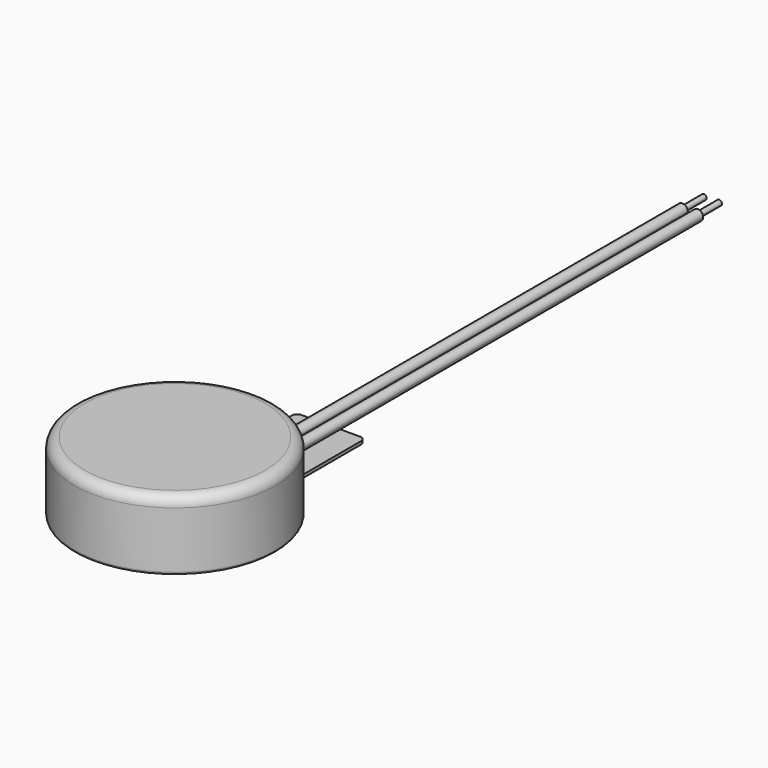
from build123d import *

# Parameters (mm, degrees)
F0_R      = 5.0038
F1_DEPTH  = 3.4544
F2_R      = 1.143
F3_DEPTH  = 0.1524
F6_DEPTH  = 1.27
F7_DEPTH  = 1.27
F8_DEPTH  = 27.94
F9_DEPTH  = 27.94
F10_R     = 0.2667
F10_R_2   = 0.13335
F11_DEPTH = 1.3335
F12_DEPTH = 1.3335
F13_R     = 0.508
F14_R     = 0.127


with BuildPart() as f1:
    # F0 (on Top) → F1 (new body)
    with BuildSketch(Plane.XY):
        with Locations((-16.2086095661, 14.8969562724)):
            Circle(F0_R)
    extrude(amount=F1_DEPTH)

    # F13
    f13_edges = [f1.edges().sort_by_distance(p)[0] for p in [
        (-21.21241, 14.896956, 3.4544),
    ]]
    fillet(f13_edges, radius=F13_R)

    # F14
    f14_edges = [f1.edges().sort_by_distance(p)[0] for p in [
        (-21.21241, 14.896956, 0),
    ]]
    fillet(f14_edges, radius=F14_R)


with BuildPart() as f3:
    # F2 (on face) → F3 (new body)
    with BuildSketch(Plane(origin=(0, 0, 0), x_dir=(1, 0, 0), z_dir=(0, 0, -1))):
        with BuildLine():
            Line((-17.9294595661, -19.2057716882), (-17.9294595661, -19.5955400716))
            ThreePointArc((-17.9294595661, -19.5955400716), (-16.2086095661, -19.9007562724), (-14.4877595661, -19.5955400716))
            Line((-14.4877595661, -19.5955400716), (-14.4877595661, -19.2057716882))
            ThreePointArc((-14.4877595661, -19.2057716882), (-14.3430605213, -18.6170461492), (-13.9419363215, -18.1624749774))
            ThreePointArc((-13.9419363215, -18.1624749774), (-16.2086095661, -10.9218562724), (-18.4752828106, -18.1624749774))
            ThreePointArc((-18.4752828106, -18.1624749774), (-18.0741586109, -18.6170461492), (-17.9294595661, -19.2057716882))
        make_face()
        with Locations((-16.2086095661, -14.8969562724)):
            Circle(F2_R, mode=Mode.SUBTRACT)
        with BuildLine():
            ThreePointArc((-14.4877595661, -19.5955400716), (-16.2086095661, -19.9007562724), (-17.9294595661, -19.5955400716))
            Line((-17.9294595661, -19.5955400716), (-17.9294595661, -24.3330562724))
            ThreePointArc((-17.9294595661, -24.3330562724), (-17.8550646885, -24.5126613948), (-17.6754595661, -24.5870562724))
            Line((-17.6754595661, -24.5870562724), (-14.7417595661, -24.5870562724))
            ThreePointArc((-14.7417595661, -24.5870562724), (-14.5621544437, -24.5126613948), (-14.4877595661, -24.3330562724))
            Line((-14.4877595661, -24.3330562724), (-14.4877595661, -19.5955400716))
        make_face()
    extrude(amount=F3_DEPTH)


with BuildPart() as f6:
    # F5 (on offset) → F6 (new body)
    with BuildSketch(Plane.XZ.offset(-20.32)):
        with BuildLine():
            ThreePointArc((-16.5896095661, 0), (-16.4010241876, 0.0781146215), (-16.3229095661, 0.2667))
            ThreePointArc((-16.3229095661, 0.2667), (-16.7781949446, 0.4552853785), (-16.5896095661, 0))
        make_face()
    extrude(amount=F6_DEPTH)

    # F5 (on offset) → F8 (join)
    with BuildSketch(Plane.XZ.offset(-20.32)):
        with BuildLine():
            ThreePointArc((-16.5896095661, 0), (-16.4010241876, 0.0781146215), (-16.3229095661, 0.2667))
            ThreePointArc((-16.3229095661, 0.2667), (-16.7781949446, 0.4552853785), (-16.5896095661, 0))
        make_face()
    extrude(amount=-F8_DEPTH)

    # F10 (on face) → F12 (cut)
    with BuildSketch(Plane(origin=(0, 48.26, 0), x_dir=(-1, 0, 0), z_dir=(0, 1, 0))):
        with Locations((16.5896095661, 0.2667)):
            Circle(F10_R)
        with Locations((16.5896095661, 0.2667)):
            Circle(F10_R_2, mode=Mode.SUBTRACT)
    extrude(amount=-F12_DEPTH, mode=Mode.SUBTRACT)


with BuildPart() as f7:
    # F5 (on offset) → F7 (new body)
    with BuildSketch(Plane.XZ.offset(-20.32)):
        with BuildLine():
            ThreePointArc((-15.5609095661, 0.2667), (-16.0161949446, 0.4552853785), (-15.8276095661, 0))
            ThreePointArc((-15.8276095661, 0), (-15.6390241876, 0.0781146215), (-15.5609095661, 0.2667))
        make_face()
    extrude(amount=F7_DEPTH)

    # F5 (on offset) → F9 (join)
    with BuildSketch(Plane.XZ.offset(-20.32)):
        with BuildLine():
            ThreePointArc((-15.5609095661, 0.2667), (-16.0161949446, 0.4552853785), (-15.8276095661, 0))
            ThreePointArc((-15.8276095661, 0), (-15.6390241876, 0.0781146215), (-15.5609095661, 0.2667))
        make_face()
    extrude(amount=-F9_DEPTH)

    # F10 (on face) → F11 (cut)
    with BuildSketch(Plane(origin=(0, 48.26, 0), x_dir=(-1, 0, 0), z_dir=(0, 1, 0))):
        with Locations((15.8276095661, 0.2667)):
            Circle(F10_R)
        with Locations((15.8276095661, 0.2667)):
            Circle(F10_R_2, mode=Mode.SUBTRACT)
    extrude(amount=-F11_DEPTH, mode=Mode.SUBTRACT)


solid = Compound([f1.part, f3.part, f6.part, f7.part])
